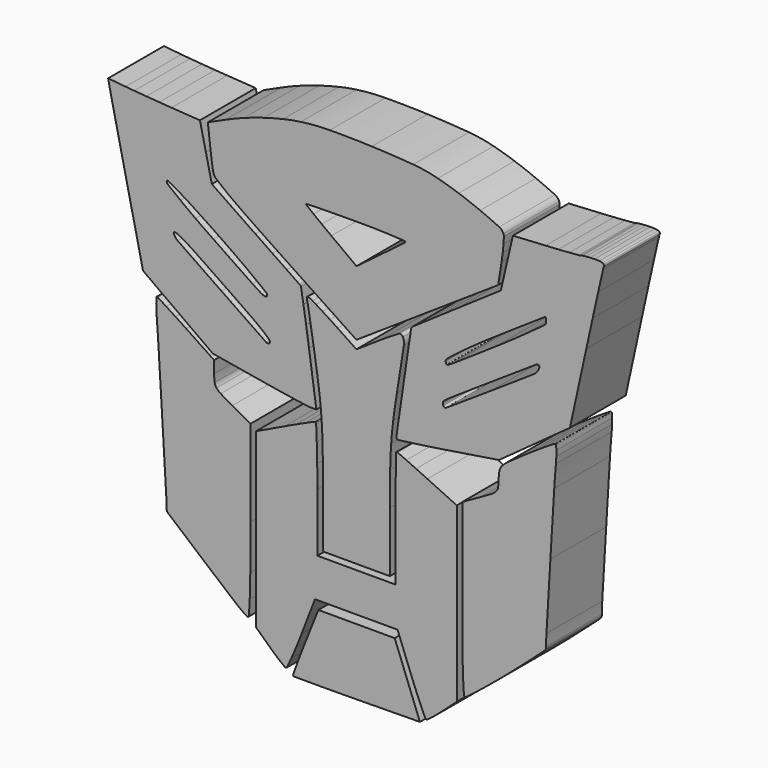
from build123d import *

# Parameters (mm, degrees)
F1_DEPTH = 25


# Not quite as in the source:
# - ends of sketch curves that miss each other by under 0.0002 mm in the source are joined


with BuildPart() as f1:
    # F0 (on Front) → F1 (new body)
    with BuildSketch(Plane.XZ):
        with BuildLine():
            ThreePointArc((-21.6550193961, -8.5406851493), (-23.6484928824, -9.4746006161), (-25.6375644051, -10.417855151))
            Line((-25.6375644051, -10.417855151), (-35.887564, -15.308075))
            Line((-35.887564, -15.308075), (-35.887564, -46.239371))
            Line((-35.887564, -46.239371), (-35.887564, -77.170666))
            Line((-35.887564, -77.170666), (-30.930405, -81.807508))
            ThreePointArc((-30.930405, -81.807508), (-29.9584582919, -82.7031449088), (-28.9732502681, -83.5841733044))
            ThreePointArc((-28.9732502681, -83.5841733044), (-28.0926396843, -84.3429562713), (-27.1956280653, -85.082278081))
            ThreePointArc((-27.1956280653, -85.082278081), (-26.4383950342, -85.6844513131), (-25.6733329969, -86.276645996))
            ThreePointArc((-25.6733329969, -86.276645996), (-25.4391547386, -86.4012895485), (-25.177389, -86.44435))
            ThreePointArc((-25.177389, -86.44435), (-24.924536283, -86.3704803587), (-24.7512179772, -86.1721070106))
            ThreePointArc((-24.7512179772, -86.1721070106), (-23.9708863493, -84.4745945867), (-23.2006555017, -82.7724752237))
            ThreePointArc((-23.2006555017, -82.7724752237), (-22.3180716015, -80.7616805071), (-21.4692575235, -78.736399195))
            ThreePointArc((-21.4692575235, -78.736399195), (-20.505028919, -76.3453141972), (-19.5656702869, -73.9443498895))
            Line((-19.5656702869, -73.9443498895), (-14.749808, -61.44435))
            Line((-14.749808, -61.44435), (0.049604, -61.44435))
            Line((0.049604, -61.44435), (14.849016, -61.44435))
            Line((14.849016, -61.44435), (19.671829, -73.94435))
            ThreePointArc((19.671829, -73.94435), (20.6105962381, -76.3447829525), (21.5712594947, -78.7365372057))
            ThreePointArc((21.5712594947, -78.7365372057), (22.4125966733, -80.7608390954), (23.283783574, -82.7724751882))
            ThreePointArc((23.283783574, -82.7724751882), (24.046866777, -84.4885222647), (24.8179486429, -86.2009901618))
            ThreePointArc((24.8179486429, -86.2009901618), (24.9708398445, -86.3782356102), (25.195385, -86.44435))
            ThreePointArc((25.195385, -86.44435), (25.4311150603, -86.4057871408), (25.6422689648, -86.2941189535))
            ThreePointArc((25.6422689648, -86.2941189535), (26.4195925866, -85.698632158), (27.1908057736, -85.0952527137))
            ThreePointArc((27.1908057736, -85.0952527137), (28.1004631808, -84.3619535951), (28.9960723919, -83.6115614588))
            ThreePointArc((28.9960723919, -83.6115614588), (30.0057731162, -82.738006763), (31.0042816903, -81.8516806556))
            Line((31.0042816903, -81.8516806556), (36.112436, -77.259011))
            Line((36.112436, -77.259011), (36.112436, -46.286461))
            Line((36.112436, -46.286461), (36.112436, -15.31391))
            Line((36.112436, -15.31391), (25.571121, -10.37913))
            ThreePointArc((25.571121, -10.37913), (23.5356700463, -9.4301344179), (21.4972641842, -8.4875026001))
            ThreePointArc((21.4972641842, -8.4875026001), (19.7463894098, -7.6863932827), (17.9915788638, -6.8939423035))
            ThreePointArc((17.9915788638, -6.8939423035), (16.4527059512, -6.2046445453), (14.9130399264, -5.517120165))
            ThreePointArc((14.9130399264, -5.517120165), (14.7459094718, -5.4627440849), (14.571121, -5.44435))
            ThreePointArc((14.571121, -5.44435), (14.4400201169, -5.4977452667), (14.383530774, -5.6275429946))
            ThreePointArc((14.383530774, -5.6275429946), (14.3139489278, -8.6202895141), (14.2471745414, -11.61309999))
            ThreePointArc((14.2471745414, -11.61309999), (14.1847188358, -15.0023348234), (14.1453983858, -18.3919170032))
            ThreePointArc((14.1453983858, -18.3919170032), (14.1206753353, -22.4180997634), (14.1124360002, -26.44435))
            Line((14.1124360002, -26.44435), (14.112436, -47.44435))
            Line((14.112436, -47.44435), (0.112436, -47.44435))
            Line((0.112436, -47.44435), (-13.887564, -47.44435))
            Line((-13.887564, -47.44435), (-13.887564, -26.44435))
            ThreePointArc((-13.887564, -26.44435), (-13.9010376036, -22.4194918168), (-13.941453004, -18.394814))
            ThreePointArc((-13.941453004, -18.394814), (-14.0057275251, -15.0096079325), (-14.1078771469, -11.6253330053))
            ThreePointArc((-14.1078771469, -11.6253330053), (-14.2164680758, -8.6940637511), (-14.3324339341, -5.7630769973))
            ThreePointArc((-14.3324339341, -5.7630769973), (-14.4270173201, -5.5606848109), (-14.6375640024, -5.4859939569))
            ThreePointArc((-14.6375640024, -5.4859939569), (-14.9125952668, -5.5263369871), (-15.1759281688, -5.6153626181))
            ThreePointArc((-15.1759281688, -5.6153626181), (-16.6779420132, -6.2816498746), (-18.1781890584, -6.9519058697))
            ThreePointArc((-18.1781890584, -6.9519058697), (-19.9194422123, -7.7400849565), (-21.6550193961, -8.5406851493))
        make_face()
    extrude(amount=F1_DEPTH)


with BuildPart() as f1b:
    # F0 (on Front) → F1, piece 2 (new body)
    with BuildSketch(Plane.XZ):
        with BuildLine():
            ThreePointArc((-17.6946806478, 32.7360990566), (-17.5720989891, 32.0449197212), (-17.4272056796, 31.358071073))
            ThreePointArc((-17.4272056796, 31.358071073), (-17.2614390204, 30.5790809799), (-17.1182136786, 29.795633054))
            ThreePointArc((-17.1182136786, 29.795633054), (-16.7171075838, 27.3950018431), (-16.3200245925, 24.9937019025))
            ThreePointArc((-16.3200245925, 24.9937019025), (-15.8532195297, 22.1333021129), (-15.3936932072, 19.271723967))
            ThreePointArc((-15.3936932072, 19.271723967), (-14.8913776494, 16.0989894545), (-14.3949965928, 12.9253210633))
            ThreePointArc((-14.3949965928, 12.9253210633), (-13.7085944575, 8.2683265335), (-13.095638916, 3.6010970104))
            ThreePointArc((-13.095638916, 3.6010970104), (-12.6731980769, -0.2650649183), (-12.3581850718, -4.1414590048))
            ThreePointArc((-12.3581850718, -4.1414590048), (-12.1261138218, -8.3531376977), (-11.9965830847, -12.5692160016))
            ThreePointArc((-11.9965830847, -12.5692160016), (-11.9148184602, -18.4466947394), (-11.887564, -24.324679))
            Line((-11.887564, -24.324679), (-11.887564, -45.44435))
            Line((-11.887564, -45.44435), (0.112436, -45.44435))
            Line((0.112436, -45.44435), (12.112436, -45.44435))
            Line((12.112436, -45.44435), (12.112436, -23.890793))
            ThreePointArc((12.112436, -23.890793), (12.1385770541, -17.8487398454), (12.2169919953, -11.807139))
            ThreePointArc((12.2169919953, -11.807139), (12.3417255499, -7.6261900586), (12.571103446, -3.4496749626))
            ThreePointArc((12.571103446, -3.4496749626), (12.881603776, 0.3203477421), (13.303460317, 4.0795389597))
            ThreePointArc((13.303460317, 4.0795389597), (13.9199856204, 8.621693178), (14.6124365413, 13.1528939126))
            ThreePointArc((14.6124365413, 13.1528939126), (15.8680121902, 21.0306955329), (17.0926815511, 28.9133609155))
            ThreePointArc((17.0926815511, 28.9133609155), (17.1163804607, 30.2564071453), (16.7822229086, 31.5574349628))
            ThreePointArc((16.7822229086, 31.5574349628), (16.1309324071, 32.1702698816), (15.2415507803, 32.076748371))
            ThreePointArc((15.2415507803, 32.076748371), (11.9009255773, 30.0387822588), (8.6149850196, 27.9137699705))
            Line((8.6149850196, 27.9137699705), (0.117533, 22.258829))
            Line((0.117533, 22.258829), (-6.635015, 26.743309))
            ThreePointArc((-6.635015, 26.743309), (-8.0087975579, 27.6501700687), (-9.3875990964, 28.5493818513))
            ThreePointArc((-9.3875990964, 28.5493818513), (-10.7283749192, 29.4126847367), (-12.0744021258, 30.2677768006))
            ThreePointArc((-12.0744021258, 30.2677768006), (-13.2289441694, 30.9916911035), (-14.3875927144, 31.7090144642))
            ThreePointArc((-14.3875927144, 31.7090144642), (-15.0230016623, 32.0864866687), (-15.6697730871, 32.4441408365))
            ThreePointArc((-15.6697730871, 32.4441408365), (-16.3633435795, 32.802871989), (-17.065558763, 33.144371503))
            ThreePointArc((-17.065558763, 33.144371503), (-17.2959084997, 33.1891113891), (-17.5197271354, 33.1186282191))
            ThreePointArc((-17.5197271354, 33.1186282191), (-17.6651448802, 32.9538633242), (-17.6946806478, 32.7360990566))
        make_face()
    extrude(amount=F1_DEPTH)


with BuildPart() as f1c:
    # F0 (on Front) → F1, piece 3 (new body)
    with BuildSketch(Plane.XZ):
        with BuildLine():
            ThreePointArc((-71.582900791, 11.0856789608), (-71.5041054764, 9.6950376898), (-71.4056497965, 8.3056499379))
            ThreePointArc((-71.4056497965, 8.3056499379), (-71.1137251421, 4.3452759792), (-70.8553786459, 0.3825699606))
            ThreePointArc((-70.8553786459, 0.3825699606), (-70.1524703664, -11.2038308529), (-69.4558428324, -22.79061099))
            ThreePointArc((-69.4558428324, -22.79061099), (-68.7119355079, -35.2395496955), (-67.9703682147, -47.6886280128))
            ThreePointArc((-67.9703682147, -47.6886280128), (-67.908269788, -49.0815095974), (-67.887564, -50.475621))
            ThreePointArc((-67.887564, -50.475621), (-67.7825288887, -50.9525071875), (-67.4868619784, -51.3411379746))
            ThreePointArc((-67.4868619784, -51.3411379746), (-61.0835784643, -56.7703228135), (-54.6762363454, -62.1947172262))
            ThreePointArc((-54.6762363454, -62.1947172262), (-48.7654501935, -67.1778050255), (-42.8378447197, -72.1408736641))
            ThreePointArc((-42.8378447197, -72.1408736641), (-41.0360996728, -73.536166576), (-39.1375639081, -74.7965988499))
            ThreePointArc((-39.1375639081, -74.7965988499), (-38.698399658, -74.813540473), (-38.4549193696, -74.4476589718))
            ThreePointArc((-38.4549193696, -74.4476589718), (-38.2750554052, -71.7828892476), (-38.1414712548, -69.1153990308))
            ThreePointArc((-38.1414712548, -69.1153990308), (-38.002065926, -64.8388795979), (-37.9376853334, -60.5605729979))
            ThreePointArc((-37.9376853334, -60.5605729979), (-37.9000951407, -52.5750423199), (-37.887564, -44.589433))
            Line((-37.887564, -44.589433), (-37.887564, -13.616482))
            Line((-37.887564, -13.616482), (-44.387564, -9.981475))
            ThreePointArc((-44.387564, -9.981475), (-46.4756151393, -8.790577889), (-48.5433120175, -7.5646810289))
            ThreePointArc((-48.5433120175, -7.5646810289), (-49.3513985165, -6.9769899117), (-50.048120618, -6.2607755063))
            ThreePointArc((-50.048120618, -6.2607755063), (-50.4793316279, -5.5555957165), (-50.7027329195, -4.759785989))
            ThreePointArc((-50.7027329195, -4.759785989), (-50.8413030857, -3.4069992311), (-50.887564, -2.047921))
            Line((-50.887564, -2.047921), (-50.887564, 2.250625))
            Line((-50.887564, 2.250625), (-60.879259, 8.903138))
            ThreePointArc((-60.879259, 8.903138), (-62.8110750122, 10.1827399957), (-64.748944884, 11.4531551779))
            ThreePointArc((-64.748944884, 11.4531551779), (-66.4191843245, 12.5335759371), (-68.0974581801, 13.6014737145))
            ThreePointArc((-68.0974581801, 13.6014737145), (-69.5622168301, 14.5237727885), (-71.0288300989, 15.4431198419))
            ThreePointArc((-71.0288300989, 15.4431198419), (-71.2169810251, 15.5269608219), (-71.420959, 15.55565))
            ThreePointArc((-71.420959, 15.55565), (-71.5645123239, 15.4970310384), (-71.6260026322, 15.3546839926))
            ThreePointArc((-71.6260026322, 15.3546839926), (-71.6400234618, 14.3903711097), (-71.64333926, 13.4259619995))
            ThreePointArc((-71.64333926, 13.4259619995), (-71.6269915227, 12.255462248), (-71.582900791, 11.0856789608))
        make_face()
    extrude(amount=F1_DEPTH)


with BuildPart() as f1d:
    # F0 (on Front) → F1, piece 4 (new body)
    with BuildSketch(Plane.XZ):
        with BuildLine():
            Line((-13.525401, -64.44435), (-18.186484, -76.131015))
            ThreePointArc((-18.186484, -76.131015), (-19.0752698547, -78.3804442062), (-19.9495733262, -80.6355418747))
            ThreePointArc((-19.9495733262, -80.6355418747), (-20.6752201035, -82.5552157389), (-21.3807059366, -84.4823900228))
            ThreePointArc((-21.3807059366, -84.4823900228), (-21.9841165896, -86.1641903759), (-22.5834954307, -87.8474318472))
            ThreePointArc((-22.5834954307, -87.8474318472), (-22.5930717521, -88.0086942921), (-22.5150800773, -88.1501670773))
            ThreePointArc((-22.5150800773, -88.1501670773), (-22.3676697701, -88.2488737589), (-22.1937759978, -88.2839984468))
            ThreePointArc((-22.1937759978, -88.2839984468), (-18.9289132097, -88.2959169663), (-15.6640439982, -88.3059223606))
            ThreePointArc((-15.6640439982, -88.3059223606), (-11.991307479, -88.3077215305), (-8.3186010008, -88.292757878))
            ThreePointArc((-8.3186010008, -88.292757878), (-3.9888945974, -88.2591831373), (0.3407010034, -88.2135022844))
            Line((0.3407010034, -88.2135022844), (22.863995, -87.94435))
            Line((22.863995, -87.94435), (18.352573, -76.19435))
            Line((18.352573, -76.19435), (13.841151, -64.44435))
            Line((13.841151, -64.44435), (0.157875, -64.44435))
            Line((0.157875, -64.44435), (-13.525401, -64.44435))
        make_face()
    extrude(amount=F1_DEPTH)


with BuildPart() as f1e:
    # F0 (on Front) → F1, piece 5 (new body)
    with BuildSketch(Plane.XZ):
        with BuildLine():
            ThreePointArc((64.655511238, 11.4174486429), (62.7545596548, 10.1411826277), (60.8624362461, 8.8518646414))
            ThreePointArc((60.8624362461, 8.8518646414), (57.6664880699, 6.637751952), (54.4896315539, 4.3963322221))
            ThreePointArc((54.4896315539, 4.3963322221), (53.3599317535, 3.4932096668), (52.3375828172, 2.4701481634))
            ThreePointArc((52.3375828172, 2.4701481634), (51.7584108888, 1.6266461393), (51.4110871912, 0.6642001797))
            ThreePointArc((51.4110871912, 0.6642001797), (51.1873224868, -0.6880753309), (51.112436, -2.056692))
            ThreePointArc((51.112436, -2.056692), (51.0649770863, -3.3837946461), (50.9228409625, -4.7041169946))
            ThreePointArc((50.9228409625, -4.7041169946), (50.6950747402, -5.4958074889), (50.261383622, -6.196209687))
            ThreePointArc((50.261383622, -6.196209687), (49.5586417661, -6.9131184293), (48.7460897732, -7.5026636249))
            ThreePointArc((48.7460897732, -7.5026636249), (46.6894543692, -8.7224643691), (44.6124356452, -9.9072243655))
            Line((44.6124356452, -9.9072243655), (38.112436, -13.542232))
            Line((38.112436, -13.542232), (38.112436, -44.615736))
            ThreePointArc((38.112436, -44.615736), (38.1248050267, -52.6583440478), (38.1619129987, -60.700876))
            ThreePointArc((38.1619129987, -60.700876), (38.2257635234, -64.9626825394), (38.3648623685, -69.2226970262))
            ThreePointArc((38.3648623685, -69.2226970262), (38.4982367321, -71.8309712836), (38.6817641699, -74.4361969864))
            ThreePointArc((38.6817641699, -74.4361969864), (38.9318122323, -74.7902400788), (39.3624360724, -74.7409110955))
            ThreePointArc((39.3624360724, -74.7409110955), (43.9509105671, -71.1851027863), (48.4655128913, -67.5359608683))
            ThreePointArc((48.4655128913, -67.5359608683), (53.3380642506, -63.4498453346), (58.1462412539, -59.2881712887))
            ThreePointArc((58.1462412539, -59.2881712887), (62.7763003803, -55.1976621482), (67.3870669439, -51.0854189374))
            ThreePointArc((67.3870669439, -51.0854189374), (67.9228525813, -50.3507290547), (68.112436, -49.461407))
            ThreePointArc((68.112436, -49.461407), (68.1433888531, -47.3504854771), (68.2362199771, -45.2413789987))
            ThreePointArc((68.2362199771, -45.2413789987), (68.9399389876, -33.303902195), (69.6492443183, -21.366756019))
            ThreePointArc((69.6492443183, -21.366756019), (70.3329594607, -9.9896039794), (71.0266862738, 1.3869419832))
            ThreePointArc((71.0266862738, 1.3869419832), (71.2962677149, 5.3482499077), (71.6181676643, 9.3056499415))
            ThreePointArc((71.6181676643, 9.3056499415), (71.7095382631, 10.5028056835), (71.7731290146, 11.7017579994))
            ThreePointArc((71.7731290146, 11.7017579994), (71.7952386392, 12.7098972138), (71.7780892253, 13.7181330082))
            ThreePointArc((71.7780892253, 13.7181330082), (71.7379807356, 14.5061649345), (71.6752330302, 15.2927180028))
            ThreePointArc((71.6752330302, 15.2927180028), (71.58284513, 15.4769078413), (71.3902860055, 15.5502722077))
            ThreePointArc((71.3902860055, 15.5502722077), (71.1102159236, 15.5094101243), (70.8518738027, 15.3937883156))
            ThreePointArc((70.8518738027, 15.3937883156), (69.4125874275, 14.4899199406), (67.9768673989, 13.5803973731))
            ThreePointArc((67.9768673989, 13.5803973731), (66.3104659657, 12.5077116103), (64.655511238, 11.4174486429))
        make_face()
    extrude(amount=F1_DEPTH)


with BuildPart() as f1f:
    # F0 (on Front) → F1, piece 6 (new body)
    with BuildSketch(Plane.XZ):
        with BuildLine():
            ThreePointArc((81.2173680585, 78.1887305187), (80.9111024816, 78.1346342816), (80.6124361652, 78.0478965277))
            ThreePointArc((80.6124361652, 78.0478965277), (80.2453883314, 77.9447286015), (79.8683370231, 77.8881597327))
            ThreePointArc((79.8683370231, 77.8881597327), (78.1690400887, 77.7437979137), (76.4692829885, 77.6049591436))
            ThreePointArc((76.4692829885, 77.6049591436), (74.4691742869, 77.4517320931), (72.4680659887, 77.3121651707))
            ThreePointArc((72.4680659887, 77.3121651707), (70.1905288319, 77.1664455388), (67.9123389834, 77.0313132918))
            Line((67.9123389834, 77.0313132918), (56.212242, 76.364588))
            Line((56.212242, 76.364588), (54.050018, 67.007514))
            Line((54.050018, 67.007514), (51.887793, 57.650439))
            Line((51.887793, 57.650439), (36.250115, 46.94266))
            ThreePointArc((36.250115, 46.94266), (33.2375819113, 44.8789203314), (30.2259194946, 42.813910279))
            ThreePointArc((30.2259194946, 42.813910279), (27.6553818366, 41.0492981297), (25.0860343032, 39.2829535593))
            ThreePointArc((25.0860343032, 39.2829535593), (22.8117460358, 37.7181346041), (20.5376331729, 36.1530607488))
            ThreePointArc((20.5376331729, 36.1530607488), (20.3683717827, 36.0315766932), (20.2040261463, 35.9035208197))
            ThreePointArc((20.2040261463, 35.9035208197), (19.8635585174, 35.5024149973), (19.6915461702, 35.0052069747))
            ThreePointArc((19.6915461702, 35.0052069747), (18.3757468708, 26.1414623349), (17.0656913623, 17.2768669466))
            ThreePointArc((17.0656913623, 17.2768669466), (15.7560378048, 8.3777498744), (14.45138656, -0.5221019356))
            ThreePointArc((14.45138656, -0.5221019356), (14.4865875977, -0.9657828044), (14.7108431199, -1.3502318877))
            ThreePointArc((14.7108431199, -1.3502318877), (14.8786906595, -1.4605708598), (15.0783859867, -1.4822328969))
            ThreePointArc((15.0783859867, -1.4822328969), (17.682503762, -1.1433553833), (20.2861370037, -0.8007750277))
            ThreePointArc((20.2861370037, -0.8007750277), (23.2462857958, -0.39760875), (26.2032620484, 0.0282026727))
            ThreePointArc((26.2032620484, 0.0282026727), (29.6813409991, 0.5510232308), (33.1569189747, 1.0902191604))
            Line((33.1569189747, 1.0902191604), (51.222972, 3.936551))
            Line((51.222972, 3.936551), (63.939806, 13.155496))
            Line((63.939806, 13.155496), (76.65664, 22.37444))
            Line((76.65664, 22.37444), (82.518947, 49.215045))
            ThreePointArc((82.518947, 49.215045), (83.6560544412, 54.4047917401), (84.8000427417, 59.5930260571))
            ThreePointArc((84.8000427417, 59.5930260571), (85.7944255611, 64.066746974), (86.7980219343, 68.5384100148))
            ThreePointArc((86.7980219343, 68.5384100148), (87.6771549826, 72.4314776858), (88.558545398, 76.3240349098))
            ThreePointArc((88.558545398, 76.3240349098), (88.689189846, 76.8199563288), (88.8538339486, 77.3056500194))
            ThreePointArc((88.8538339486, 77.3056500194), (88.8893141531, 77.5853728036), (88.7941128283, 77.8507788876))
            ThreePointArc((88.7941128283, 77.8507788876), (88.5771582723, 78.0863963188), (88.2957131674, 78.2392804838))
            ThreePointArc((88.2957131674, 78.2392804838), (87.7679470504, 78.3813880716), (87.2255019913, 78.4483578346))
            ThreePointArc((87.2255019913, 78.4483578346), (86.3477229255, 78.4786028755), (85.4694250023, 78.4767028883))
            ThreePointArc((85.4694250023, 78.4767028883), (84.6942000932, 78.4547977482), (83.9194100331, 78.4208293595))
            ThreePointArc((83.9194100331, 78.4208293595), (83.1850751059, 78.3761923249), (82.4516760087, 78.3181749019))
            ThreePointArc((82.4516760087, 78.3181749019), (81.8339902305, 78.2585236659), (81.2173680585, 78.1887305187))
        make_face()
        with BuildLine():
            ThreePointArc((65.6666797095, 37.7844198705), (65.6084659694, 37.5411591049), (65.5242047342, 37.3056496914))
            ThreePointArc((65.5242047342, 37.3056496914), (64.7810083135, 36.0746166725), (63.7164310184, 35.1079429726))
            ThreePointArc((63.7164310184, 35.1079429726), (55.9797716493, 29.9249647204), (48.224751111, 24.7694998323))
            ThreePointArc((48.224751111, 24.7694998323), (40.2587801741, 19.5061718121), (32.2818057087, 14.2595354439))
            ThreePointArc((32.2818057087, 14.2595354439), (31.6832959099, 14.1853674852), (31.2595014835, 14.6144518278))
            ThreePointArc((31.2595014835, 14.6144518278), (31.1968481313, 14.827470917), (31.1495472061, 15.0444160373))
            ThreePointArc((31.1495472061, 15.0444160373), (31.121901816, 15.2487786622), (31.1125379454, 15.45479))
            ThreePointArc((31.1125379454, 15.45479), (31.1209601573, 15.6234070354), (31.1464436453, 15.7902998676))
            ThreePointArc((31.1464436453, 15.7902998676), (31.1864884893, 15.8935862841), (31.2582694448, 15.9779614702))
            ThreePointArc((31.2582694448, 15.9779614702), (32.7789381704, 17.1853454922), (34.3632050911, 18.3079798638))
            ThreePointArc((34.3632050911, 18.3079798638), (41.6155904038, 23.1480624729), (48.8747738955, 27.9779431573))
            ThreePointArc((48.8747738955, 27.9779431573), (56.6587939516, 33.1474519474), (64.4443743698, 38.3146104426))
            ThreePointArc((64.4443743698, 38.3146104426), (64.8262431699, 38.4940790046), (65.243666, 38.55565))
            ThreePointArc((65.243666, 38.55565), (65.3846136915, 38.5290507545), (65.5061729514, 38.4529119474))
            ThreePointArc((65.5061729514, 38.4529119474), (65.6024774908, 38.3322781218), (65.6585487118, 38.1884619353))
            ThreePointArc((65.6585487118, 38.1884619353), (65.6829508292, 37.9868502136), (65.6666797095, 37.7844198705))
        make_face(mode=Mode.SUBTRACT)
        with BuildLine():
            ThreePointArc((68.0944909851, 53.6368899991), (68.107948664, 53.3544128932), (68.112436, 53.071651))
            ThreePointArc((68.112436, 53.071651), (67.9372867858, 52.3356619316), (67.4493897928, 51.7574632805))
            ThreePointArc((67.4493897928, 51.7574632805), (63.7595663672, 49.0505324838), (60.0517854372, 46.3682513914))
            ThreePointArc((60.0517854372, 46.3682513914), (55.0246355008, 42.8085266445), (49.9495549175, 39.3174761217))
            ThreePointArc((49.9495549175, 39.3174761217), (42.4319816235, 34.2456583416), (34.8918428345, 29.2074492489))
            ThreePointArc((34.8918428345, 29.2074492489), (34.1166287011, 28.7035601406), (33.3310567515, 28.2159764098))
            ThreePointArc((33.3310567515, 28.2159764098), (32.9867344132, 28.055221659), (32.6159190968, 27.97217914))
            ThreePointArc((32.6159190968, 27.97217914), (32.394310638, 28.020278776), (32.2472754281, 28.1929181708))
            ThreePointArc((32.2472754281, 28.1929181708), (32.1464512369, 28.537366849), (32.112436, 28.894653))
            ThreePointArc((32.112436, 28.894653), (32.2330019849, 29.4195834985), (32.5705332656, 29.8392986632))
            ThreePointArc((32.5705332656, 29.8392986632), (34.8820683991, 31.6472621804), (37.207925657, 33.4367634495))
            ThreePointArc((37.207925657, 33.4367634495), (40.0377005905, 35.5561669997), (42.9050719911, 37.6244220126))
            ThreePointArc((42.9050719911, 37.6244220126), (46.3710691187, 40.0501585422), (49.8624357501, 42.4392363694))
            ThreePointArc((49.8624357501, 42.4392363694), (53.2732345415, 44.7448118554), (56.6859591761, 47.0475357388))
            ThreePointArc((56.6859591761, 47.0475357388), (59.5775511893, 48.9939859094), (62.4718110921, 50.9364668625))
            ThreePointArc((62.4718110921, 50.9364668625), (65.0732627803, 52.679654162), (67.6748926761, 54.4225754835))
            ThreePointArc((67.6748926761, 54.4225754835), (67.764889833, 54.4712124763), (67.8624361248, 54.5020304183))
            ThreePointArc((67.8624361248, 54.5020304183), (67.9227731652, 54.4920787182), (67.9601603996, 54.4436861162))
            ThreePointArc((67.9601603996, 54.4436861162), (68.0042516386, 54.2749148965), (68.0389979188, 54.1039749858))
            ThreePointArc((68.0389979188, 54.1039749858), (68.0731431801, 53.8711927089), (68.0944909851, 53.6368899991))
        make_face(mode=Mode.SUBTRACT)
    extrude(amount=F1_DEPTH)


with BuildPart() as f1g:
    # F0 (on Front) → F1, piece 7 (new body)
    with BuildSketch(Plane.XZ):
        with BuildLine():
            ThreePointArc((-9.4544350059, 88.2994017785), (-14.6532515018, 88.0889089931), (-19.8269891125, 87.5371488032))
            ThreePointArc((-19.8269891125, 87.5371488032), (-23.0078270354, 87.0189983537), (-26.1623390706, 86.3592533035))
            ThreePointArc((-26.1623390706, 86.3592533035), (-29.679561229, 85.4826771247), (-33.1674670881, 84.4958892936))
            ThreePointArc((-33.1674670881, 84.4958892936), (-36.7193209952, 83.3703929604), (-40.2347719486, 82.1358838605))
            ThreePointArc((-40.2347719486, 82.1358838605), (-43.5252572447, 80.8548739374), (-46.7671768349, 79.4555036357))
            Line((-46.7671768349, 79.4555036357), (-53.146789, 76.563542))
            Line((-53.146789, 76.563542), (-52.440687, 70.309596))
            ThreePointArc((-52.440687, 70.309596), (-52.2910137578, 69.0202721598), (-52.1332440106, 67.7319139987))
            ThreePointArc((-52.1332440106, 67.7319139987), (-51.9673895166, 66.4446093196), (-51.7934512679, 65.1583719629))
            ThreePointArc((-51.7934512679, 65.1583719629), (-51.6346363886, 64.0364951107), (-51.4689336368, 62.9156149039))
            ThreePointArc((-51.4689336368, 62.9156149039), (-51.3573629217, 62.2341397278), (-51.2288789806, 61.5556500039))
            ThreePointArc((-51.2288789806, 61.5556500039), (-50.8301894117, 60.5207115116), (-50.1123562014, 59.6752727602))
            ThreePointArc((-50.1123562014, 59.6752727602), (-47.8764795256, 57.8498571569), (-45.5902017711, 56.0879773059))
            ThreePointArc((-45.5902017711, 56.0879773059), (-41.9578596582, 53.4336629421), (-38.2656274924, 50.8633097472))
            ThreePointArc((-38.2656274924, 50.8633097472), (-31.796191065, 46.4919972068), (-25.3053690496, 42.1525029254))
            Line((-25.3053690496, 42.1525029254), (0.112436, 25.249356))
            Line((0.112436, 25.249356), (25.523965, 42.152503))
            Line((25.523965, 42.152503), (50.935494, 59.05565))
            Line((50.935494, 59.05565), (52.141813, 66.777353))
            ThreePointArc((52.141813, 66.777353), (52.3667002886, 68.3053011469), (52.5645427508, 69.8369859098))
            ThreePointArc((52.5645427508, 69.8369859098), (52.7164597842, 71.2381924592), (52.8357735514, 72.6425509596))
            ThreePointArc((52.8357735514, 72.6425509596), (52.9105248992, 73.8102014528), (52.9637719214, 74.9790300029))
            ThreePointArc((52.9637719214, 74.9790300029), (52.933570409, 75.4476415998), (52.8102532717, 75.9007441043))
            ThreePointArc((52.8102532717, 75.9007441043), (52.2148984745, 76.8518155638), (51.305416131, 77.5089502834))
            ThreePointArc((51.305416131, 77.5089502834), (47.9149237415, 79.0362555371), (44.4958750705, 80.4985161693))
            ThreePointArc((44.4958750705, 80.4985161693), (40.669135567, 82.0211372377), (36.7959149998, 83.4213059995))
            ThreePointArc((36.7959149998, 83.4213059995), (33.0628156138, 84.6277748813), (29.2878688358, 85.6961263763))
            ThreePointArc((29.2878688358, 85.6961263763), (24.9066499122, 86.6441345068), (20.4587220532, 87.2006746627))
            ThreePointArc((20.4587220532, 87.2006746627), (13.0478832888, 87.7164918625), (5.6277219777, 88.0739894058))
            ThreePointArc((5.6277219777, 88.0739894058), (-1.91208732, 88.2716158093), (-9.4544350059, 88.2994017785))
        make_face()
        with BuildLine():
            ThreePointArc((17.4452849999, 62.0490929984), (17.6170290256, 61.91812509), (17.5624363456, 61.7091556121))
            ThreePointArc((17.5624363456, 61.7091556121), (17.2283263214, 61.4219456107), (16.8842129485, 61.1468000668))
            ThreePointArc((16.8842129485, 61.1468000668), (15.6792276077, 60.2194955872), (14.4727677374, 59.2941103429))
            ThreePointArc((14.4727677374, 59.2941103429), (13.0388089409, 58.1990770946), (11.6019248575, 57.1078851882))
            ThreePointArc((11.6019248575, 57.1078851882), (9.9913551024, 55.8906093701), (8.3784608597, 54.6764151868))
            Line((8.3784608597, 54.6764151868), (0.144486, 48.490166))
            Line((0.144486, 48.490166), (-8.871539, 55.152492))
            ThreePointArc((-8.871539, 55.152492), (-10.6030214211, 56.4386288069), (-12.3280828134, 57.7333652474))
            ThreePointArc((-12.3280828134, 57.7333652474), (-13.7880914294, 58.8441063212), (-15.2391068695, 59.9665701673))
            ThreePointArc((-15.2391068695, 59.9665701673), (-16.5068837838, 60.957122393), (-17.7730560982, 61.949724875))
            ThreePointArc((-17.7730560982, 61.949724875), (-17.8574196976, 62.0542983637), (-17.887564, 62.185234))
            ThreePointArc((-17.887564, 62.185234), (-17.8443292133, 62.2912560008), (-17.7392829864, 62.3368103822))
            ThreePointArc((-17.7392829864, 62.3368103822), (-15.1403208801, 62.3928827762), (-12.5413139896, 62.4468394894))
            ThreePointArc((-12.5413139896, 62.4468394894), (-9.6039591889, 62.4972770769), (-6.6663430029, 62.5290313745))
            ThreePointArc((-6.6663430029, 62.5290313745), (-3.1769788812, 62.5489947666), (0.312436, 62.55565))
            ThreePointArc((0.312436, 62.55565), (3.7710907251, 62.5405584905), (7.2294819999, 62.4952809923))
            ThreePointArc((7.2294819999, 62.4952809923), (10.0599424528, 62.4235170532), (12.8889169968, 62.3070719339))
            ThreePointArc((12.8889169968, 62.3070719339), (15.1675864214, 62.1866559049), (17.4452849999, 62.0490929984))
        make_face(mode=Mode.SUBTRACT)
    extrude(amount=F1_DEPTH)


with BuildPart() as f1h:
    # F0 (on Front) → F1, piece 8 (new body)
    with BuildSketch(Plane.XZ):
        with BuildLine():
            Line((-88.892912, 78.832388), (-88.297005, 75.944019))
            ThreePointArc((-88.297005, 75.944019), (-88.084374815, 74.9303529327), (-87.8650424691, 73.9181158967))
            ThreePointArc((-87.8650424691, 73.9181158967), (-87.040235916, 70.1737678297), (-86.214471153, 66.4296309662))
            ThreePointArc((-86.214471153, 66.4296309662), (-85.2356598684, 61.9990401573), (-84.2548287446, 57.5688960566))
            ThreePointArc((-84.2548287446, 57.5688960566), (-83.1503821714, 52.5895795483), (-82.0443320302, 47.6106189933))
            Line((-82.0443320302, 47.6106189933), (-76.387564, 22.165589))
            Line((-76.387564, 22.165589), (-63.887564, 13.17206))
            Line((-63.887564, 13.17206), (-51.387564, 4.178531))
            Line((-51.387564, 4.178531), (-34.887564, 1.380295))
            ThreePointArc((-34.887564, 1.380295), (-31.6526233386, 0.837839808), (-28.4156978732, 0.307356783))
            ThreePointArc((-28.4156978732, 0.307356783), (-25.5216468266, -0.1537428943), (-22.6252450552, -0.5998383647))
            ThreePointArc((-22.6252450552, -0.5998383647), (-20.184258814, -0.9654568767), (-17.7421530441, -1.3235213043))
            ThreePointArc((-17.7421530441, -1.3235213043), (-17.0297858085, -1.4019246855), (-16.3137129993, -1.4311458894))
            Line((-16.3137129993, -1.4311458894), (-14.239862, -1.44435))
            Line((-14.239862, -1.44435), (-16.88598, 17.044584))
            ThreePointArc((-16.88598, 17.044584), (-17.4019287213, 20.6019310254), (-17.9312491847, 24.1573129721))
            ThreePointArc((-17.9312491847, 24.1573129721), (-18.3966717311, 27.1813798961), (-18.8804479264, 30.202565012))
            ThreePointArc((-18.8804479264, 30.202565012), (-19.3164978016, 32.8646903714), (-19.7554232214, 35.5263431288))
            ThreePointArc((-19.7554232214, 35.5263431288), (-19.8253289944, 35.7193959387), (-19.9598309036, 35.8745261209))
            ThreePointArc((-19.9598309036, 35.8745261209), (-20.1314560161, 36.0062856728), (-20.3077909649, 36.1316720514))
            ThreePointArc((-20.3077909649, 36.1316720514), (-22.5856148175, 37.6891657134), (-24.8636160872, 39.2463998724))
            ThreePointArc((-24.8636160872, 39.2463998724), (-27.439623177, 41.0059064619), (-30.016777002, 42.763732997))
            ThreePointArc((-30.016777002, 42.763732997), (-33.0344296477, 44.8196732838), (-36.052920934, 46.874382097))
            Line((-36.052920934, 46.874382097), (-51.718279, 57.53323))
            Line((-51.718279, 57.53323), (-53.853233, 66.904951))
            Line((-53.853233, 66.904951), (-55.988188, 76.276672))
            Line((-55.988188, 76.276672), (-66.187876, 76.946637))
            ThreePointArc((-66.187876, 76.946637), (-68.3697136902, 77.093558352), (-70.5510559458, 77.2476607493))
            ThreePointArc((-70.5510559458, 77.2476607493), (-72.8898265588, 77.4198930797), (-75.2281289592, 77.5983695253))
            ThreePointArc((-75.2281289592, 77.5983695253), (-77.3834255383, 77.7686962148), (-79.5382550215, 77.944833741))
            ThreePointArc((-79.5382550215, 77.944833741), (-81.0897361386, 78.0792334587), (-82.6402379485, 78.2244955293))
            Line((-82.6402379485, 78.2244955293), (-88.892912, 78.832388))
        make_face()
        with BuildLine():
            ThreePointArc((-58.0264078918, 34.2622891607), (-52.6921945154, 30.6557720335), (-47.3717678888, 27.0289471624))
            ThreePointArc((-47.3717678888, 27.0289471624), (-42.5826989866, 23.7350915051), (-37.8085135006, 20.4197002826))
            ThreePointArc((-37.8085135006, 20.4197002826), (-35.5587867991, 18.7937478202), (-33.364219175, 17.0940817816))
            ThreePointArc((-33.364219175, 17.0940817816), (-32.2009246238, 16.0998528226), (-31.1027955902, 15.0340864292))
            ThreePointArc((-31.1027955902, 15.0340864292), (-30.8951476513, 14.5145037732), (-31.1114267781, 13.9984537781))
            ThreePointArc((-31.1114267781, 13.9984537781), (-31.6092818733, 13.764277501), (-32.1421119799, 13.9013540295))
            ThreePointArc((-32.1421119799, 13.9013540295), (-40.1946888899, 19.3882203361), (-48.240829822, 24.8845202603))
            ThreePointArc((-48.240829822, 24.8845202603), (-56.0999274427, 30.2717327057), (-63.9478780721, 35.6751708956))
            ThreePointArc((-63.9478780721, 35.6751708956), (-64.7761110822, 36.4441252163), (-65.3512573643, 37.4169908504))
            ThreePointArc((-65.3512573643, 37.4169908504), (-65.2811753948, 37.8744004796), (-64.8442221629, 38.0267372213))
            ThreePointArc((-64.8442221629, 38.0267372213), (-63.7951107657, 37.7186598435), (-62.8079449535, 37.2485000805))
            ThreePointArc((-62.8079449535, 37.2485000805), (-60.3915321196, 35.7964564186), (-58.0264078918, 34.2622891607))
        make_face(mode=Mode.SUBTRACT)
        with BuildLine():
            ThreePointArc((-32.29997776, 29.6707893097), (-31.9962128109, 29.2979486105), (-31.887564, 28.829463))
            ThreePointArc((-31.887564, 28.829463), (-32.0610456975, 28.4305659541), (-32.4711169921, 28.2854581118))
            ThreePointArc((-32.4711169921, 28.2854581118), (-33.1745120897, 28.4185806238), (-33.8279128311, 28.7110762832))
            ThreePointArc((-33.8279128311, 28.7110762832), (-35.506128807, 29.7450135647), (-37.1539988253, 30.8266602581))
            ThreePointArc((-37.1539988253, 30.8266602581), (-44.1477116468, 35.5663184217), (-51.1375639474, 40.3116680773))
            ThreePointArc((-51.1375639474, 40.3116680773), (-54.3603775407, 42.528403874), (-57.5577838979, 44.7816321432))
            ThreePointArc((-57.5577838979, 44.7816321432), (-60.2803292857, 46.7602470599), (-62.9672510249, 48.7869739676))
            ThreePointArc((-62.9672510249, 48.7869739676), (-65.2185113952, 50.5301565276), (-67.4566564514, 52.2901466923))
            ThreePointArc((-67.4566564514, 52.2901466923), (-67.7741849991, 52.6864282865), (-67.887564, 53.181412))
            ThreePointArc((-67.887564, 53.181412), (-67.7144489787, 53.4832613477), (-67.3664938215, 53.4862693175))
            ThreePointArc((-67.3664938215, 53.4862693175), (-65.2056361993, 52.253329249), (-63.0608120084, 50.992703986))
            ThreePointArc((-63.0608120084, 50.992703986), (-60.2167849635, 49.2559994643), (-57.4095576228, 47.4604195764))
            ThreePointArc((-57.4095576228, 47.4604195764), (-53.6378345165, 44.969070544), (-49.8875643375, 42.4455435031))
            ThreePointArc((-49.8875643375, 42.4455435031), (-46.425871501, 40.0695022636), (-42.9878660285, 37.6593139597))
            ThreePointArc((-42.9878660285, 37.6593139597), (-40.0648449489, 35.5540180466), (-37.1750635824, 33.403323552))
            ThreePointArc((-37.1750635824, 33.403323552), (-34.7320937734, 31.5441445346), (-32.29997776, 29.6707893097))
        make_face(mode=Mode.SUBTRACT)
    extrude(amount=F1_DEPTH)


solid = Compound([f1.part, f1b.part, f1c.part, f1d.part, f1e.part, f1f.part, f1g.part, f1h.part])
